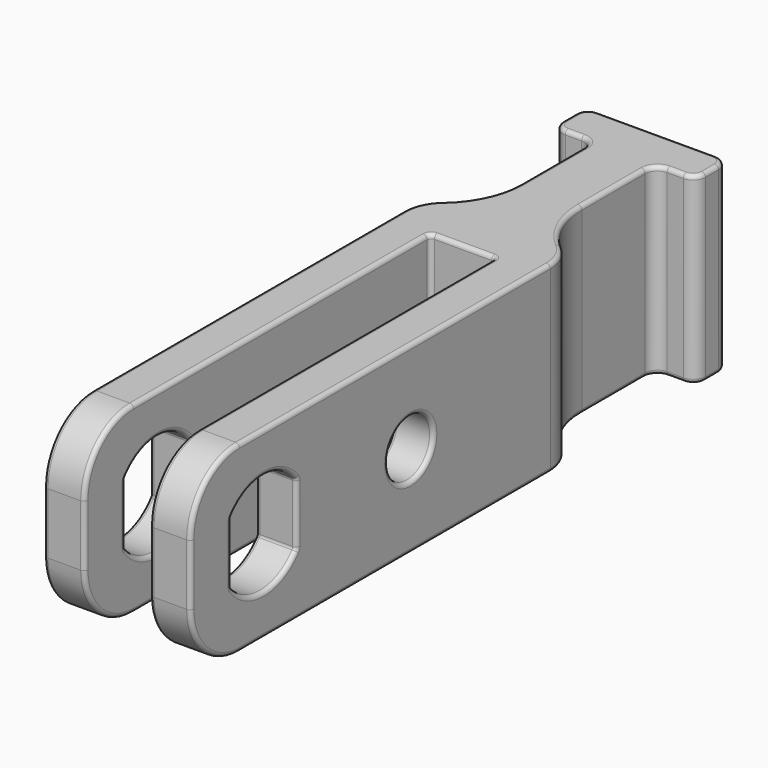
from build123d import *

# Parameters (mm, degrees)
F0_W        = 10
F0_H        = 10
F0_H_2      = 25
F0_W_2      = 15
F0_H_3      = 9.5
F0_H_4      = 40
F0_H_5      = 5
F1_DEPTH    = 45
F2_R        = 15
F4_DEPTH    = 36.001
F5_T1_DEPTH = 45
F6_R        = 10
F7_R        = 3
F8_R        = 1
F9_R        = 7
F10_DEPTH   = 36.0010001
F11_R       = 1


# Not quite as in the source:
# - a fillet or chamfer that OpenCascade refuses, or shapes differently, is made with other operations: its cross-section is extruded or revolved along the edge and cut away or added


with BuildPart() as f1:
    # F0 (on Top) → F1 (new body)
    with BuildSketch(Plane.XY):
        with Locations((-13, -17.5)):
            Rectangle(F0_W, F0_H)
        with Locations((-13, 0)):
            Rectangle(F0_W, F0_H_2)
        Polygon((-18, 12.5), (-8, 12.5), (-8, 83), (-8, 83.5), (-7.5, 83.5), (-7.5, 93), (-18, 93), align=None)
        with Locations((0, 88.25)):
            Rectangle(F0_W_2, F0_H_3)
        with Locations((0, 113)):
            Rectangle(F0_W_2, F0_H_4)
        Polygon((8, 83), (8, 12.5), (18, 12.5), (18, 93), (7.5, 93), (7.5, 83.5), (8, 83.5), align=None)
        with Locations((13, 0)):
            Rectangle(F0_W, F0_H_2)
        with Locations((13, -17.5)):
            Rectangle(F0_W, F0_H)
        with Locations((0, 135.5)):
            Rectangle(F0_W_2, F0_H_5)
        Polygon((7.5, 138), (7.5, 133), (17.5, 133), (17.5, 143), (-17.5, 143), (-17.5, 133), (-7.5, 133), (-7.5, 138), align=None)
    extrude(amount=F1_DEPTH)

    # F2
    f2_edges = [f1.edges().sort_by_distance(p)[0] for p in [
        (-13, -22.5, 45),
        (-13, -22.5, 0),
        (13, -22.5, 45),
        (13, -22.5, 0),
    ]]
    fillet(f2_edges, radius=F2_R)

    # F3 (on face) → F4 (cut, through all)
    with BuildSketch(Plane.YZ.offset(18)):
        with BuildLine():
            Line((10, 15), (10, 30))
            ThreePointArc((10, 30), (0, 35), (-10, 30))
            Line((-10, 30), (-10, 15))
            ThreePointArc((-10, 15), (0, 10), (10, 15))
        make_face()
    extrude(amount=-F4_DEPTH, mode=Mode.SUBTRACT)

    # F5: fillet of radius 20 on 2 edges, made by hand

    # F5_s2 → F5_t1 (join)
    with BuildSketch(Plane.XY):
        with BuildLine():
            ThreePointArc((-18, 93), (-10.3244359627, 100.3527651408), (-7.5, 110.5997159068))
            Line((-7.5, 110.5997159068), (-7.5, 93))
            Line((-7.5, 93), (-18, 93))
        make_face()
        with BuildLine():
            ThreePointArc((18, 93), (10.3244359627, 100.3527651408), (7.5, 110.5997159068))
            Line((7.5, 110.5997159068), (7.5, 93))
            Line((7.5, 93), (18, 93))
        make_face()
    extrude(amount=F5_T1_DEPTH)

    # F6
    f6_edges = [f1.edges().sort_by_distance(p)[0] for p in [
        (18, 93, 22.5),
        (-18, 93, 22.5),
    ]]
    fillet(f6_edges, radius=F6_R)

    # F7
    f7_edges = [f1.edges().sort_by_distance(p)[0] for p in [
        (-7.5, 133, 22.5),
        (-17.5, 133, 22.5),
        (-17.5, 143, 22.5),
        (7.5, 133, 22.5),
        (17.5, 133, 22.5),
        (17.5, 143, 22.5),
    ]]
    fillet(f7_edges, radius=F7_R)

    # F8
    f8_edges = [f1.edges().sort_by_distance(p)[0] for p in [
        (-18, -22.5, 22.5),
        (-13, -22.5, 15),
        (-13, -22.5, 30),
        (-8, -22.5, 22.5),
        (8, -22.5, 22.5),
        (13, -22.5, 15),
        (13, -22.5, 30),
        (18, -22.5, 22.5),
        (18, 0, 10),
        (13, 10, 15),
        (8, 0, 10),
        (13, -10, 15),
        (18, -10, 22.5),
        (8, -10, 22.5),
        (13, -10, 30),
        (18, 0, 35),
        (8, 0, 35),
        (13, 10, 30),
        (-8, -10, 22.5),
        (-13, -10, 15),
        (-18, -10, 22.5),
        (-13, -10, 30),
        (-8, 0, 35),
        (-18, 0, 35),
        (-13, 10, 30),
        (-8, 10, 22.5),
        (-18, 10, 22.5),
        (-13, 10, 15),
        (-8, 83.5, 22.5),
        (8, 83.5, 22.5),
        (0, 83.5, 0),
        (0, 83.5, 45),
        (7.5, 120.299858, 0),
        (8.37868, 132.12132, 0),
        (9.334098, 102.233116, 0),
        (12.5, 133, 0),
        (17.082951, 91.98499, 0),
        (16.62132, 133.87868, 0),
        (18, 40.150845, 0),
        (17.5, 138, 0),
        (16.62132, 142.12132, 0),
        (8, 38, 0),
        (0, 143, 0),
        (-16.62132, 142.12132, 0),
        (-8, 38, 0),
        (-17.5, 138, 0),
        (-16.62132, 133.87868, 0),
        (-18, 40.150845, 0),
        (-12.5, 133, 0),
        (-17.082951, 91.98499, 0),
        (-8.37868, 132.12132, 0),
        (-9.334098, 102.233116, 0),
        (-7.5, 120.299858, 0),
        (7.5, 120.299858, 45),
        (8.37868, 132.12132, 45),
        (9.334098, 102.233116, 45),
        (12.5, 133, 45),
        (17.082951, 91.98499, 45),
        (16.62132, 133.87868, 45),
        (18, -18.106602, 4.393398),
        (18, 40.150845, 45),
        (18, -18.106602, 40.606602),
        (18, 10, 22.5),
        (17.5, 138, 45),
        (8, -18.106602, 4.393398),
        (16.62132, 142.12132, 45),
        (8, -18.106602, 40.606602),
        (8, 38, 45),
        (8, 10, 22.5),
        (0, 143, 45),
        (-16.62132, 142.12132, 45),
        (-8, -18.106602, 4.393398),
        (-8, -18.106602, 40.606602),
        (-8, 38, 45),
        (-8, 0, 10),
        (-17.5, 138, 45),
        (-18, -18.106602, 4.393398),
        (-16.62132, 133.87868, 45),
        (-18, 40.150845, 45),
        (-18, -18.106602, 40.606602),
        (-18, 0, 10),
        (-12.5, 133, 45),
        (-17.082951, 91.98499, 45),
        (-8.37868, 132.12132, 45),
        (-9.334098, 102.233116, 45),
        (-7.5, 120.299858, 45),
    ]]
    fillet(f8_edges, radius=F8_R)

    # F9 (on face) → F10 (cut, through all)
    with BuildSketch(Plane(origin=(-18, 0, 0), x_dir=(0, -1, 0), z_dir=(-1, 0, 0))):
        with Locations((-45, 22.5)):
            Circle(F9_R)
    extrude(amount=-F10_DEPTH, mode=Mode.SUBTRACT)

    # F11
    f11_edges = [f1.edges().sort_by_distance(p)[0] for p in [
        (8, 52, 22.5),
        (13, 38, 22.5),
        (18, 52, 22.5),
        (-18, 52, 22.5),
        (-13, 38, 22.5),
        (-8, 52, 22.5),
    ]]
    fillet(f11_edges, radius=F11_R)


solid = f1.part
